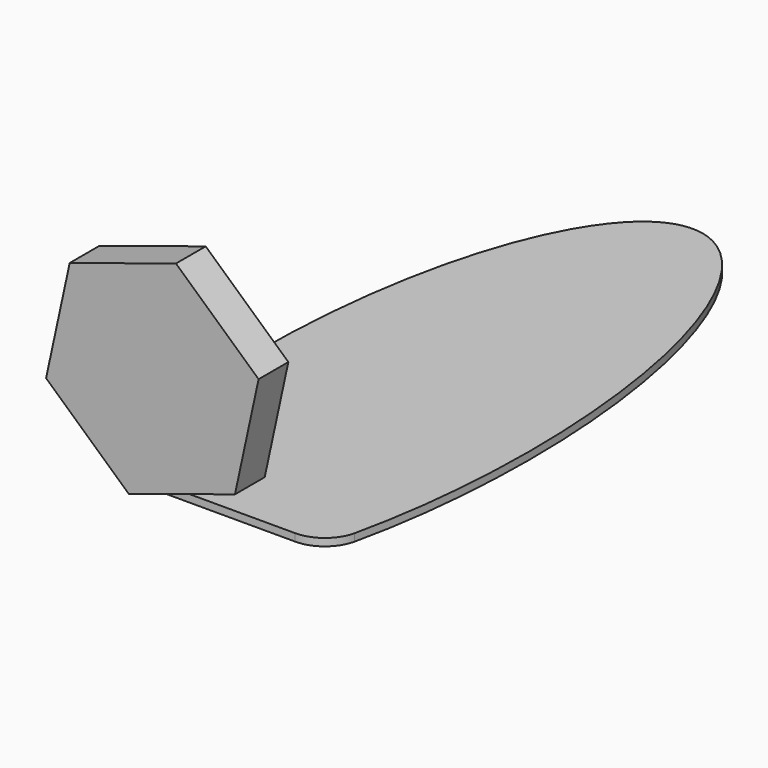
from build123d import *

# Parameters (mm, degrees)
F1_DEPTH = 5
F4_DEPTH = 1
F5_R     = 5


with BuildPart() as f1:
    # F0 (on Front) → F1 (new body)
    with BuildSketch(Plane.XZ):
        Polygon((14.2836181896, 4.5802021149), (3.1752377088, 14.6600772676), (-11.1083804808, 10.0798751527), (-14.2836181896, -4.5802021149), (-3.1752377088, -14.6600772676), (11.1083804808, -10.0798751527), align=None)
    extrude(amount=F1_DEPTH)

    # F3 (on offset) → F4 (join)
    with BuildSketch(Plane.XY.offset(-15)):
        with BuildLine():
            add(Edge.make_bspline(
                [(20.7579379474, -2.0610693128), (42.8052881355, 78.0521397261), (6.1978475941, 78.0521397261)],
                knots=[4.0660546316, 4.0660546316, 4.0660546316, 6.2831853072, 6.2831853072, 6.2831853072], degree=2, weights=[1, 0.4459460837, 1]))
            add(Edge.make_bspline(
                [(6.1978475941, 78.0521397261), (-30.4095929472, 78.0521397261), (-8.3622427591, -2.0610693128)],
                knots=[0, 0, 0, 2.2171306756, 2.2171306756, 2.2171306756], degree=2, weights=[1, 0.4459460837, 1]))
            Line((-8.3622427591, -2.0610693128), (20.7579379474, -2.0610693128))
        make_face()
    extrude(amount=F4_DEPTH)

    # F5
    f5_edges = [f1.edges().sort_by_distance(p)[0] for p in [
        (-8.362243, -2.061069, -14.5),
        (20.757938, -2.061069, -14.5),
    ]]
    fillet(f5_edges, radius=F5_R)


solid = f1.part
